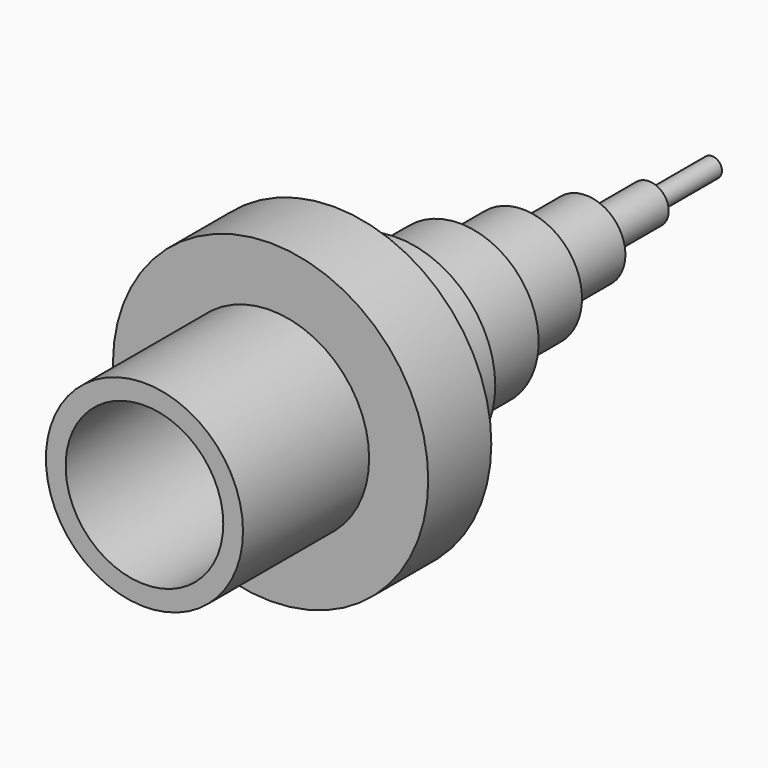
from build123d import *

# Parameters (mm, degrees)
F0_R      = 40
F1_DEPTH  = 20
F2_R      = 25
F5_DEPTH  = 40
F3_R      = 25
F6_DEPTH  = 25.4
F7_DEPTH  = 20
F8_R      = 20
F9_DEPTH  = 20
F10_R     = 15
F11_DEPTH = 20
F12_R     = 10
F13_DEPTH = 20
F14_R     = 5
F15_DEPTH = 20
F16_R     = 2.5
F17_DEPTH = 20
F18_R     = 20
F19_DEPTH = 40


# Not quite as in the source:
# - the program builds the solid bodies; features that only make, move or delete a surface that nothing else refers to are left out


with BuildPart() as f1:
    # F0 (on Front) → F1 (new body)
    with BuildSketch(Plane.XZ):
        Circle(F0_R)
    extrude(amount=F1_DEPTH)

    # F2 (on face) → F5 (join)
    with BuildSketch(Plane.XZ.offset(20)):
        Circle(F2_R)
    extrude(amount=F5_DEPTH)

    # F3 (on face) → F6 (join)
    with BuildSketch(Plane.XZ):
        Circle(F3_R)
    extrude(amount=F6_DEPTH)

    # F3 (on face) → F7 (join)
    with BuildSketch(Plane.XZ):
        Circle(F3_R)
    extrude(amount=-F7_DEPTH)

    # F8 (on face) → F9 (join)
    with BuildSketch(Plane(origin=(0, 20, 0), x_dir=(-1, 0, 0), z_dir=(0, 1, 0))):
        Circle(F8_R)
    extrude(amount=F9_DEPTH)

    # F10 (on face) → F11 (join)
    with BuildSketch(Plane(origin=(0, 40, 0), x_dir=(-1, 0, 0), z_dir=(0, 1, 0))):
        Circle(F10_R)
    extrude(amount=F11_DEPTH)

    # F12 (on face) → F13 (join)
    with BuildSketch(Plane(origin=(0, 60, 0), x_dir=(-1, 0, 0), z_dir=(0, 1, 0))):
        Circle(F12_R)
    extrude(amount=F13_DEPTH)

    # F14 (on face) → F15 (join)
    with BuildSketch(Plane(origin=(0, 80, 0), x_dir=(-1, 0, 0), z_dir=(0, 1, 0))):
        Circle(F14_R)
    extrude(amount=F15_DEPTH)

    # F16 (on face) → F17 (join)
    with BuildSketch(Plane(origin=(0, 100, 0), x_dir=(-1, 0, 0), z_dir=(0, 1, 0))):
        Circle(F16_R)
    extrude(amount=F17_DEPTH)

    # F18 (on face) → F19 (cut)
    with BuildSketch(Plane.XZ.offset(60)):
        Circle(F18_R)
    extrude(amount=-F19_DEPTH, mode=Mode.SUBTRACT)


solid = f1.part
